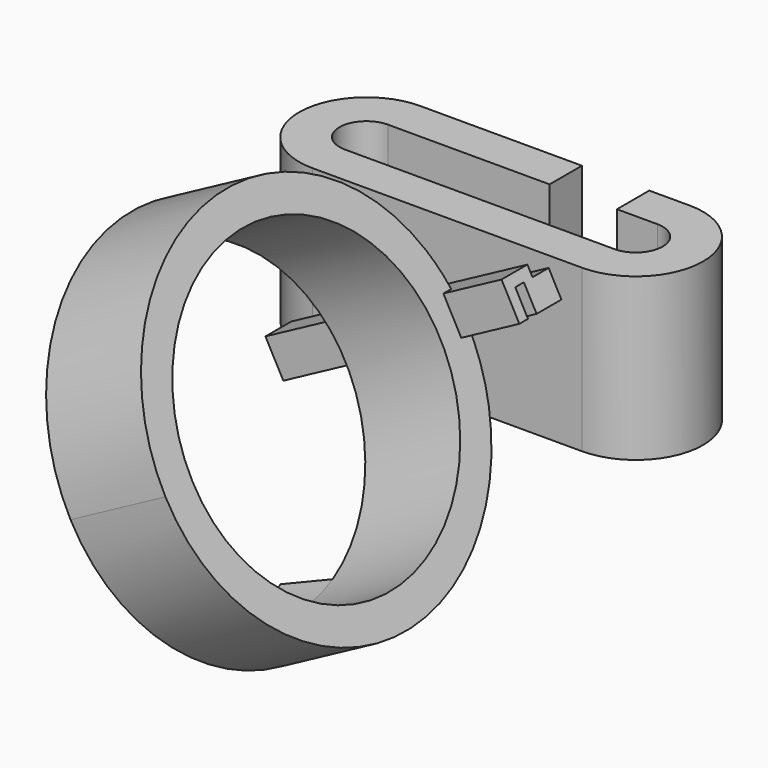
from build123d import *

# Parameters (mm, degrees)
F1_DEPTH       = 12
F5_DEPTH       = 19.9
F7_R           = 11.5
F8_DEPTH       = 8
F11_ANGLE_BACK = 20
F11_ANGLE      = 40


with BuildPart() as f1:
    # F0 (on Top) → F1 (new body)
    with BuildSketch(Plane.XY):
        with BuildLine():
            Line((0, 0), (-20, 0))
            ThreePointArc((-20, 0), (-22, 2), (-20, 4))
            Line((-20, 4), (-8, 4))
            Line((-8, 4), (-8, 7))
            Line((-8, 7), (-20, 7))
            ThreePointArc((-20, 7), (-25, 2), (-20, -3))
            Line((-20, -3), (0, -3))
            ThreePointArc((0, -3), (5, 2), (0, 7))
            Line((0, 7), (-3, 7))
            Line((-3, 7), (-3, 4))
            Line((-3, 4), (0, 4))
            ThreePointArc((0, 4), (2, 2), (0, 0))
        make_face()
    extrude(amount=F1_DEPTH)

    # F4 (on line) → F5 (join)
    with BuildSketch(Plane(origin=(-14.7844431916, 0, -7.9443702008), x_dir=(0, -1, 0), z_dir=(-0.8808807435, 0, -0.4733382677))):
        Polygon((3, 11.0186671228), (3, 9.0186671228), (5.3, 9.0186671228), (5.3, 11.0186671228), (6.1, 11.0186671228), (6.1, 9.0186671228), (6.9, 9.0186671228), (6.9, 11.8186671228), (4.5, 11.8186671228), (4.5, 11.0186671228), align=None)
    extrude(amount=-F5_DEPTH)

    # F7 (on offset) → F8 (join)
    with BuildSketch(Plane(origin=(-1.5712320387, 0, -0.8442961852), x_dir=(0, -1, 0), z_dir=(-0.8808807435, 0, -0.4733382677))):
        with BuildLine():
            ThreePointArc((34, 9.6230288318), (22.5099800796, 23.3961911411), (6.9, 14.5616521217))
            Line((6.9, 14.5616521217), (6.9, 4.6844055418))
            ThreePointArc((6.9, 4.6844055418), (22.5099800796, -4.1501334776), (34, 9.6230288318))
        make_face()
        with Locations((20, 9.6230288318)):
            Circle(F7_R, mode=Mode.SUBTRACT)
        with BuildLine():
            Line((6.9, 4.6844055418), (6.9, 14.5616521217))
            ThreePointArc((6.9, 14.5616521217), (6, 9.6230288318), (6.9, 4.6844055418))
        make_face()
    extrude(amount=F8_DEPTH)

    # F10 (on offset) → F11 (revolve)
    with BuildSketch(Plane.XZ.offset(20), mode=Mode.PRIVATE) as f11_sk:
        Polygon((-6.7922217721, -8.029286104), (-7.7298357056, -6.2843900851), (-11.4623919126, -7.7224527269), align=None)
        Polygon((-21.8758338022, 11.6569236308), (-18.6166158629, 13.9758670161), (-19.5542297964, 15.720763035), align=None)
    revolve(f11_sk.sketch.rotate(Axis((-15.3602525801, -20, 2.6705470646), (-0.8808807435, 0, -0.4733382677)), -F11_ANGLE_BACK), axis=Axis((-15.3602525801, -20, 2.6705470646), (-0.8808807435, 0, -0.4733382677)), revolution_arc=F11_ANGLE)


solid = f1.part
